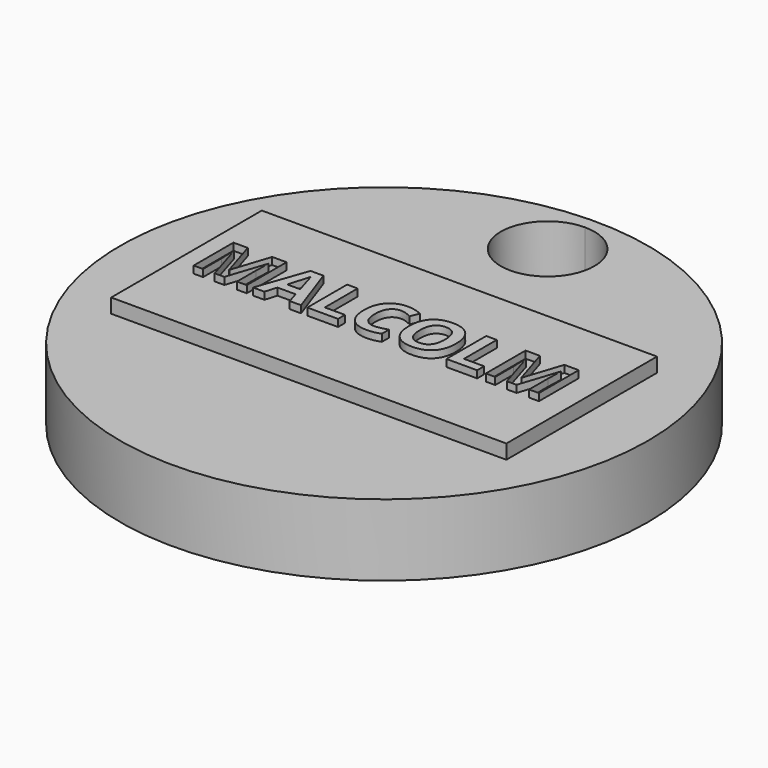
from build123d import *

# Parameters (mm, degrees)
F0_R          = 46.2666790195
F1_DEPTH      = 25.4
F3_DEPTH      = 25.4
F5_R          = 46.80588018
F6_DEPTH      = 12.7
F8_DEPTH      = 25.4
F9_W          = 70.0839459896
F9_H          = 33.3876311779
F10_DEPTH     = 2.54
F11_TEXT_SIZE = 12.3472222222
F12_DEPTH     = 1.27
F13_SCALE     = 0.45


# Not quite as in the source:
# - Text() gives the source's letters only with a copy of the font that has no kerning and outlines rounded to 1/6400 em; it was checked with that copy


with BuildPart() as f1:
    # F0 (on Top) → F1 (new body)
    with BuildSketch(Plane.XY):
        with Locations((0, 6.418844685)):
            Circle(F0_R)
    extrude(amount=F1_DEPTH)

    # F2 (on face) → F3 (cut)
    with BuildSketch(Plane.XY.offset(25.4)):
        with BuildLine():
            ThreePointArc((37.1231685655, -15.0906437155), (30.343750569, -5.3586201635), (18.8653619688, -8.3451542637))
            Line((18.8653619688, -8.3451542637), (34.6309947273, -21.8361331673))
            ThreePointArc((34.6309947273, -21.8361331673), (36.4802019001, -18.6862159365), (37.1231685655, -15.0906437155))
        make_face()
        with BuildLine():
            Line((34.6309947273, -21.8361331673), (18.8653619688, -8.3451542637))
            ThreePointArc((18.8653619688, -8.3451542637), (20.0026888962, -22.9734600947), (34.6309947273, -21.8361331673))
        make_face()
    extrude(amount=-F3_DEPTH, mode=Mode.SUBTRACT)


with BuildPart() as f6:
    # F5 (on Top) → F6 (new body)
    with BuildSketch(Plane.XY):
        Circle(F5_R)
    extrude(amount=F6_DEPTH)

    # F7 (on face) → F8 (cut)
    with BuildSketch(Plane.XY.offset(12.7)):
        with BuildLine():
            ThreePointArc((0, 44.5332311488), (-8.288097421, 36.2451337278), (0, 27.9570363068))
            Line((0, 27.9570363068), (0, 44.5332311488))
        make_face()
        with BuildLine():
            Line((0, 44.5332311488), (0, 27.9570363068))
            ThreePointArc((0, 27.9570363068), (5.8605698895, 30.3845638383), (8.288097421, 36.2451337278))
            ThreePointArc((8.288097421, 36.2451337278), (5.8605698895, 42.1057036173), (0, 44.5332311488))
        make_face()
    extrude(amount=-F8_DEPTH, mode=Mode.SUBTRACT)

    # F9 (on face) → F10 (join)
    with BuildSketch(Plane.XY.offset(12.7)):
        Rectangle(F9_W, F9_H)
    extrude(amount=F10_DEPTH)

    # F11 (on face) → F12 (join)
    with BuildSketch(Plane.XY.offset(15.24)):
        with Locations((-31.6926034372, -3.9836447274)):
            Text('MALCOLM', F11_TEXT_SIZE, font='Open Sans', font_style=FontStyle.BOLD, text_align=(TextAlign.LEFT, TextAlign.BOTTOM))
    extrude(amount=F12_DEPTH)


with BuildPart() as f6_1:
    # F13: moved
    add(f6.part.scale(F13_SCALE))


solid = f6_1.part
